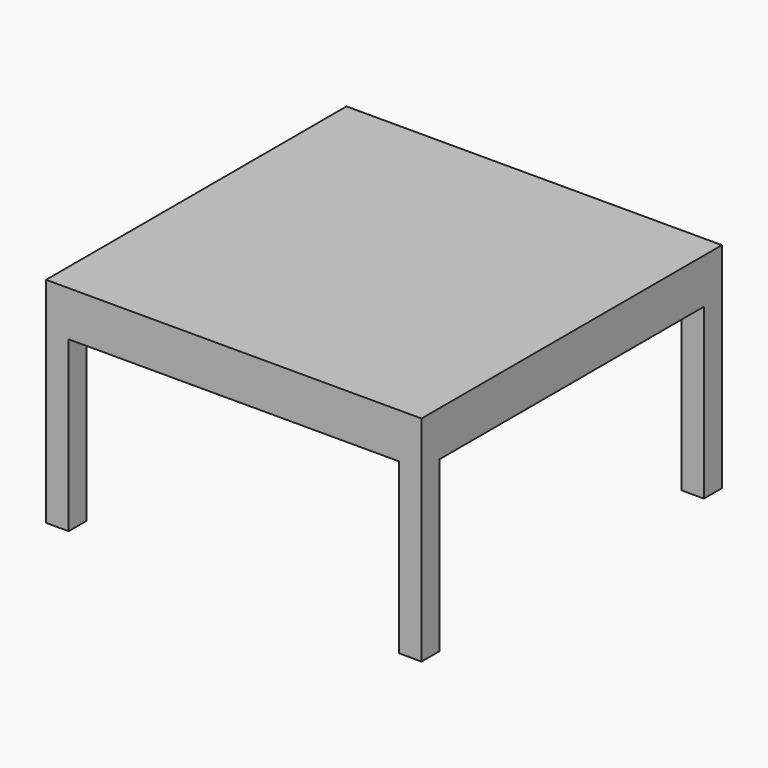
from build123d import *

# Parameters (mm, degrees)
F0_W            = 1000
F0_H            = 1000
F1_DEPTH        = 120
F2_W            = 60
F2_H            = 60
F3_DEPTH        = 450
F3_COPIES_COUNT = 4


# Not quite as in the source:
# - a pattern or mirror of a feature is missing from the dataset's text; its kind, count and spacing are read off the source's solid


with BuildPart() as f1:
    # F0 (on Top) → F1 (new body)
    with BuildSketch(Plane.XY):
        Rectangle(F0_W, F0_H)
    extrude(amount=F1_DEPTH)

    # F2 (on face) → F3 (join)
    with BuildSketch(Plane(origin=(0, 0, 0), x_dir=(1, 0, 0), z_dir=(0, 0, -1))):
        with Locations((-470, 470)):
            Rectangle(F2_W, F2_H)
    f3 = extrude(amount=F3_DEPTH)

    # F3_copies: F3 ×4 about axis
    f3_copies_axis = Axis((0, 0, 0), (0, 0, 1))
    for i in range(1, F3_COPIES_COUNT):
        add(f3.rotate(f3_copies_axis, i * 360 / F3_COPIES_COUNT))


solid = f1.part
